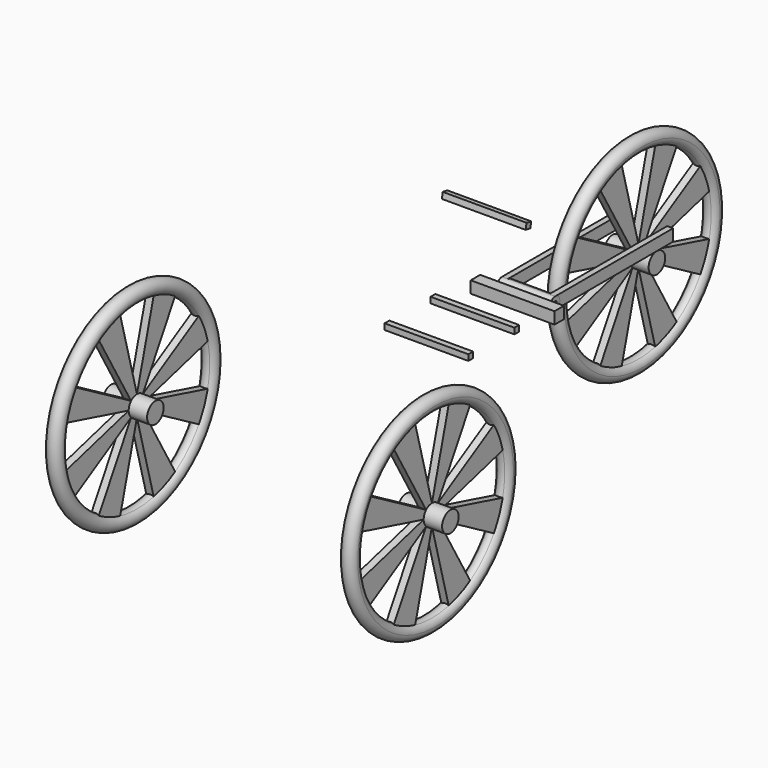
from build123d import *

# Parameters (mm, degrees)
F4_DEPTH  = 175.001
F9_W      = 40
F9_H      = 80
F10_DEPTH = 900
F11_DEPTH = 100
F13_DEPTH = 360
F14_DEPTH = 360
F15_W     = 80
F15_H     = 80
F16_DEPTH = 284
F15_W_2   = 40
F15_H_2   = 40


with BuildPart() as f1:
    # F0 (on Top) → F1 (revolve)
    with BuildSketch(Plane.XY):
        with BuildLine():
            ThreePointArc((-25, -616.6987298108), (-25, -703.3012701892), (50, -660))
            ThreePointArc((50, -660), (43.3012701892, -635), (25, -616.6987298108))
            ThreePointArc((25, -616.6987298108), (0, -610), (-25, -616.6987298108))
        make_face()
    revolve(axis=Axis((6.2885098159, 0, 0), (-1, 0, 0)))


with BuildPart() as f2:
    # F0 (on Top) → F2 (revolve)
    with BuildSketch(Plane.XY):
        with BuildLine():
            ThreePointArc((-25, -616.6987298108), (0, -610), (25, -616.6987298108))
            Line((25, -616.6987298108), (25, -70))
            Line((25, -70), (150, -70))
            Line((150, -70), (150, 0))
            Line((150, 0), (-150, 0))
            Line((-150, 0), (-150, -70))
            Line((-150, -70), (-25, -70))
            Line((-25, -70), (-25, -616.6987298108))
        make_face()
    revolve(axis=Axis((0, 0, 0), (1, 0, 0)))

    # F3 (on face) → F4 (cut, through all)
    with BuildSketch(Plane(origin=(-25, 0, 0), x_dir=(0, -1, 0), z_dir=(-1, 0, 0))):
        with BuildLine():
            Line((-142.0444833082, 600.1172286411), (0, 70))
            Line((0, 70), (142.0444833082, 600.1172286411))
            ThreePointArc((142.0444833082, 600.1172286411), (0, 616.6987298108), (-142.0444833082, 600.1172286411))
        make_face()
        with BuildLine():
            Line((323.9063445017, 524.7875792564), (49.4974746831, 49.4974746831))
            Line((49.4974746831, 49.4974746831), (524.7875792564, 323.9063445016))
            ThreePointArc((524.7875792564, 323.9063445016), (436.0718537983, 436.0718537983), (323.9063445017, 524.7875792564))
        make_face()
        with BuildLine():
            Line((600.1172286411, 142.0444833082), (70, 0))
            Line((70, 0), (600.1172286411, -142.0444833082))
            ThreePointArc((600.1172286411, -142.0444833082), (612.5393277132, -71.5045128285), (616.6987298108, 0))
            ThreePointArc((616.6987298108, 0), (612.5393277132, 71.5045128285), (600.1172286411, 142.0444833082))
        make_face()
        with BuildLine():
            Line((524.7875792564, -323.9063445016), (49.4974746831, -49.4974746831))
            Line((49.4974746831, -49.4974746831), (323.9063445016, -524.7875792564))
            ThreePointArc((323.9063445016, -524.7875792564), (436.0718537983, -436.0718537983), (524.7875792564, -323.9063445017))
        make_face()
        with BuildLine():
            Line((142.0444833082, -600.1172286411), (0, -70))
            Line((0, -70), (-142.0444833082, -600.1172286411))
            ThreePointArc((-142.0444833082, -600.1172286411), (0, -616.6987298108), (142.0444833082, -600.1172286411))
        make_face()
        with BuildLine():
            Line((-323.9063445016, -524.7875792564), (-49.4974746831, -49.4974746831))
            Line((-49.4974746831, -49.4974746831), (-524.7875792564, -323.9063445017))
            ThreePointArc((-524.7875792564, -323.9063445016), (-436.0718537983, -436.0718537983), (-323.9063445016, -524.7875792564))
        make_face()
        with BuildLine():
            Line((-600.1172286411, -142.0444833082), (-70, 0))
            Line((-70, 0), (-600.1172286411, 142.0444833082))
            ThreePointArc((-600.1172286411, 142.0444833082), (-616.6987298108, 0), (-600.1172286411, -142.0444833082))
        make_face()
        with BuildLine():
            Line((-524.7875792564, 323.9063445017), (-49.4974746831, 49.4974746831))
            Line((-49.4974746831, 49.4974746831), (-323.9063445017, 524.7875792564))
            ThreePointArc((-323.9063445016, 524.7875792564), (-436.0718537983, 436.0718537983), (-524.7875792564, 323.9063445016))
        make_face()
    extrude(amount=-F4_DEPTH, mode=Mode.SUBTRACT)


with BuildPart() as f6_1:
    # F6: instance of F1
    add(f1.part.mirror(Plane.XZ.offset(1500)))


with BuildPart() as f6_2:
    # F6: instance of F2
    add(f2.part.mirror(Plane.XZ.offset(1500)))


with BuildPart() as f6_1_1:
    # F7: moved
    add(f6_1.part.moved(Location((1000, 0, 0))))


with BuildPart() as f6_2_1:
    # F7: moved
    add(f6_2.part.moved(Location((1000, 0, 0))))


with BuildPart() as f8_1:
    # F8: instance of F6_1
    add(f6_1_1.part.mirror(Plane.YZ))


with BuildPart() as f8_2:
    # F8: instance of F6_2
    add(f6_2_1.part.mirror(Plane.YZ))


with BuildPart() as f10:
    # F9 (on Front) → F10 (new body)
    with BuildSketch(Plane.XZ):
        with Locations((160, 135)):
            Rectangle(F9_W, F9_H)
    extrude(amount=F10_DEPTH)

    # F11 (add): a face of the model
    f11_faces = [f10.faces().sort_by_distance(p)[0] for p in [
        (160, 0, 135),
    ]]
    extrude(f11_faces, amount=F11_DEPTH)


with BuildPart() as f10b:
    # F9 (on Front) → F10, piece 2 (new body)
    with BuildSketch(Plane.XZ):
        with Locations((-160, 135)):
            Rectangle(F9_W, F9_H)
    extrude(amount=F10_DEPTH)

    # F11#2 (add): a face of the model
    f11_2_faces = [f10b.faces().sort_by_distance(p)[0] for p in [
        (-160, 0, 135),
    ]]
    extrude(f11_2_faces, amount=F11_DEPTH)


with BuildPart() as f13:
    # F12 (on face) → F13 (new body, through all)
    with BuildSketch(Plane.YZ.offset(180)):
        with BuildLine():
            Line((-900, 147.5), (-900, 175))
            ThreePointArc((-900, 175), (-940, 135), (-900, 95))
            Line((-900, 95), (-900, 122.5))
            ThreePointArc((-900, 122.5), (-912.5, 135), (-900, 147.5))
        make_face()
        with BuildLine():
            ThreePointArc((-900, 95), (-871.7157287525, 106.7157287525), (-860, 135))
            ThreePointArc((-860, 135), (-871.7157287525, 163.2842712475), (-900, 175))
            Line((-900, 175), (-900, 147.5))
            ThreePointArc((-900, 147.5), (-891.1611652352, 143.8388347648), (-887.5, 135))
            ThreePointArc((-887.5, 135), (-891.1611652352, 126.1611652352), (-900, 122.5))
            Line((-900, 122.5), (-900, 95))
        make_face()
    extrude(amount=-F13_DEPTH)


with BuildPart() as f14_tool:
    # F12 (on face) → F14 (new body, through all)
    with BuildSketch(Plane.YZ.offset(180)):
        with BuildLine():
            ThreePointArc((-900, 95), (-871.7157287525, 106.7157287525), (-860, 135))
            ThreePointArc((-860, 135), (-871.7157287525, 163.2842712475), (-900, 175))
            Line((-900, 175), (-900, 147.5))
            ThreePointArc((-900, 147.5), (-891.1611652352, 143.8388347648), (-887.5, 135))
            ThreePointArc((-887.5, 135), (-891.1611652352, 126.1611652352), (-900, 122.5))
            Line((-900, 122.5), (-900, 95))
        make_face()
        with BuildLine():
            ThreePointArc((-887.5, 135), (-891.1611652352, 143.8388347648), (-900, 147.5))
            Line((-900, 147.5), (-900, 122.5))
            ThreePointArc((-900, 122.5), (-891.1611652352, 126.1611652352), (-887.5, 135))
        make_face()
    extrude(amount=-F14_DEPTH)


with BuildPart() as f10_1:
    add(f10.part)

    # F14: cut by f14_tool
    add(f14_tool.part, mode=Mode.SUBTRACT)


with BuildPart() as f10b_1:
    add(f10b.part)

    # F14: cut by f14_tool
    add(f14_tool.part, mode=Mode.SUBTRACT)


with BuildPart() as f16:
    # F15 (on Right) → F16 (new body, symmetric)
    with BuildSketch(Plane.YZ):
        with Locations((-995, 135)):
            Rectangle(F15_W, F15_H)
    extrude(amount=F16_DEPTH, both=True)


with BuildPart() as f16b:
    # F15 (on Right) → F16, piece 2 (new body, symmetric)
    with BuildSketch(Plane.YZ):
        with Locations((-1355, 195)):
            Rectangle(F15_W_2, F15_H_2)
    extrude(amount=F16_DEPTH, both=True)


with BuildPart() as f16c:
    # F15 (on Right) → F16, piece 3 (new body, symmetric)
    with BuildSketch(Plane.YZ):
        with Locations((-1745, 195)):
            Rectangle(F15_W_2, F15_H_2)
    extrude(amount=F16_DEPTH, both=True)


with BuildPart() as f16d:
    # F15 (on Right) → F16, piece 4 (new body, symmetric)
    with BuildSketch(Plane.YZ):
        Polygon((-1272.3068959168, 799.1513074579), (-1279.2528230234, 759.7589973374), (-1239.8605129029, 752.8130702308), (-1232.9145857963, 792.2053803512), align=None)
    extrude(amount=F16_DEPTH, both=True)


solid = Compound([f1.part, f2.part, f6_1_1.part, f6_2_1.part, f8_1.part, f8_2.part, f13.part, f10_1.part, f10b_1.part, f16.part, f16b.part, f16c.part, f16d.part])
